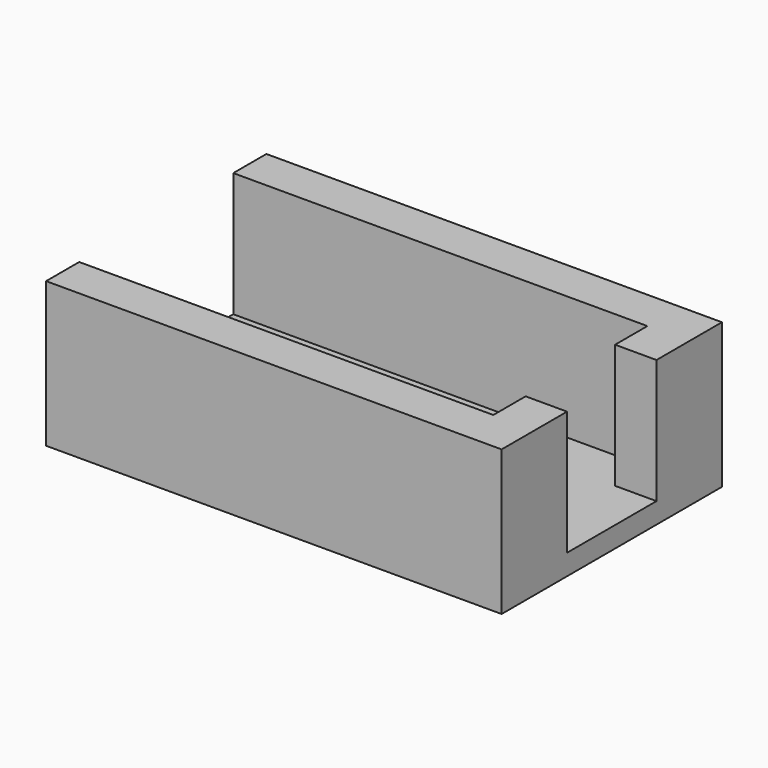
from build123d import *

# Parameters (mm, degrees)
F0_W     = 10
F0_H     = 2
F1_DEPTH = 6
F2_W     = 22
F2_H     = 13.3
F3_DEPTH = 1


with BuildPart() as f1:
    # F0 (on Top) → F1 (new body)
    with BuildSketch(Plane.XY):
        Polygon((-5, 4.65), (5, 4.65), (5, 2.7), (7, 2.7), (7, 4.85), (7, 6.65), (5, 6.65), (-5, 6.65), align=None)
        with Locations((-10, 5.65)):
            Rectangle(F0_W, F0_H)
    extrude(amount=F1_DEPTH)



with BuildPart() as f1b:
    # F0 (on Top) → F1, piece 2 (new body)
    with BuildSketch(Plane.XY):
        Polygon((5, -4.65), (-5, -4.65), (-5, -6.65), (5, -6.65), (7, -6.65), (7, -4.85), (7, -2.7), (5, -2.7), align=None)
        with Locations((-10, -5.65)):
            Rectangle(F0_W, F0_H)
    extrude(amount=F1_DEPTH)


with BuildPart() as f1_1:
    add(f1.part)

    add(f1b.part)  # F3 merges F1b
    # F2 (on Top) → F3 (join)
    with BuildSketch(Plane.XY):
        with Locations((-4, 0)):
            Rectangle(F2_W, F2_H)
    extrude(amount=-F3_DEPTH)


solid = f1_1.part
